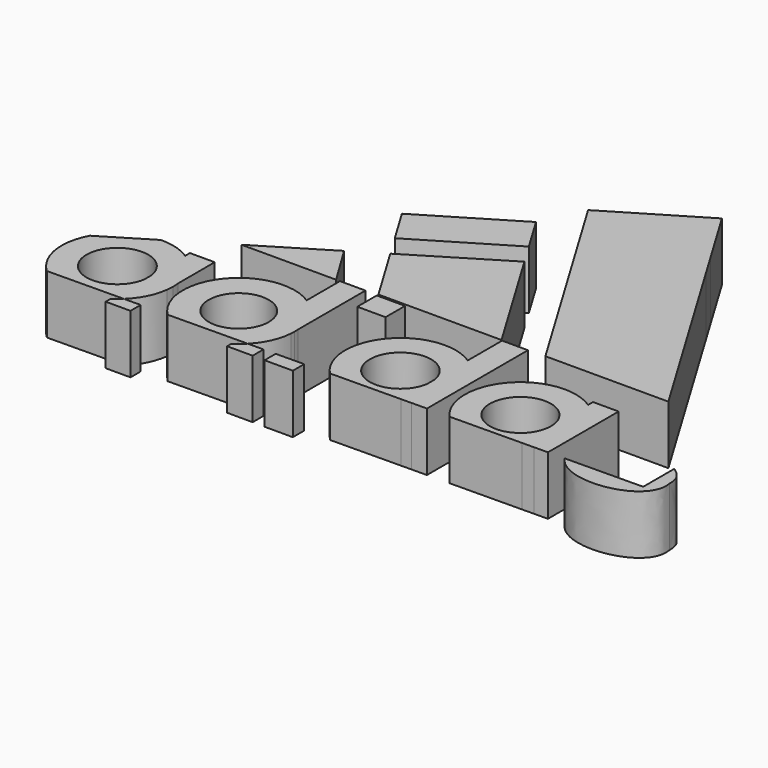
from build123d import *

# Parameters (mm, degrees)
F1_DEPTH = 7.62
F0_R     = 3.9071612502
F0_R_2   = 3.9693222288
F0_W     = 3.6783010967
F0_H     = 3.1684441492


with BuildPart() as f1:
    # F0 (on Top) → F1 (new body)
    with BuildSketch(Plane.XY):
        Polygon((-54.6120963991, 18.8028495759), (-57.9414791113, 24.2596925711), (-66.9205742951, 18.8028495759), align=None)
    extrude(amount=F1_DEPTH)


with BuildPart() as f1b:
    # F0 (on Top) → F1, piece 2 (new body)
    with BuildSketch(Plane.XY):
        Polygon((-58.4635436535, 34.3171171844), (-55.6590456115, 29.6528524318), (-43.8780021033, 36.7234046998), (-46.6844625771, 41.399564594), align=None)
    extrude(amount=F1_DEPTH)


with BuildPart() as f1c:
    # F0 (on Top) → F1, piece 3 (new body)
    with BuildSketch(Plane.XY):
        Polygon((-42.1554631157, 33.8532884785), (-53.8949323829, 26.718890265), (-49.2192299373, 18.9425560391), (-33.2065857947, 18.9425560391), align=None)
    extrude(amount=F1_DEPTH)


with BuildPart() as f1d:
    # F0 (on Top) → F1, piece 4 (new body)
    with BuildSketch(Plane.XY):
        with BuildLine():
            ThreePointArc((-69.8677301407, 13.3297108985), (-71.8363877974, 14.2310348582), (-73.9834488266, 14.5105465515))
            Line((-73.9834488266, 14.5105465515), (-80.197720877, 10.7339625846))
            ThreePointArc((-80.197720877, 10.7339625846), (-80.9859151306, 6.0900592734), (-78.7530233725, 1.9426163816))
            Line((-78.7530233725, 1.9426163816), (-69.8677301407, 2.0325591908))
            Line((-69.8677301407, 2.0325591908), (-69.8677301407, 6.657484785))
            ThreePointArc((-69.8677301407, 6.657484785), (-77.8484436742, 7.2651901282), (-69.8677301407, 7.8728954714))
            Line((-69.8677301407, 7.8728954714), (-69.8677301407, 13.3297108985))
        make_face()
        with BuildLine():
            Line((-69.8677301407, 14.1047984362), (-69.8677301407, 13.3297108985))
            ThreePointArc((-69.8677301407, 13.3297108985), (-67.6845522307, 11.0979247886), (-66.6428804398, 8.1547878725))
            Line((-66.6428804398, 8.1547878725), (-66.6428804398, 14.1047984362))
            Line((-66.6428804398, 14.1047984362), (-69.8677301407, 14.1047984362))
        make_face()
        with BuildLine():
            ThreePointArc((-66.6428804398, 8.1547878725), (-67.6845522307, 11.0979247886), (-69.8677301407, 13.3297108985))
            Line((-69.8677301407, 13.3297108985), (-69.8677301407, 7.8728954714))
            ThreePointArc((-69.8677301407, 7.8728954714), (-69.833040775, 7.5699224451), (-69.821455358, 7.2651901282))
            ThreePointArc((-69.821455358, 7.2651901282), (-69.833040775, 6.9604578114), (-69.8677301407, 6.657484785))
            Line((-69.8677301407, 6.657484785), (-69.8677301407, 2.0325591908))
            Line((-69.8677301407, 2.0325591908), (-68.810137273, 2.0432648447))
            ThreePointArc((-68.810137273, 2.0432648447), (-67.3537989415, 4.0229796207), (-66.6428804398, 6.375592384))
            Line((-66.6428804398, 6.375592384), (-66.6428804398, 8.1547878725))
        make_face()
        with BuildLine():
            ThreePointArc((-66.5880714472, 7.2651901282), (-66.6017866739, 7.7108324097), (-66.6428804398, 8.1547878725))
            Line((-66.6428804398, 8.1547878725), (-66.6428804398, 6.375592384))
            ThreePointArc((-66.6428804398, 6.375592384), (-66.6017866739, 6.8195478467), (-66.5880714472, 7.2651901282))
        make_face()
        with BuildLine():
            ThreePointArc((-69.821455358, 7.2651901282), (-69.833040775, 7.5699224451), (-69.8677301407, 7.8728954714))
            Line((-69.8677301407, 7.8728954714), (-69.8677301407, 6.657484785))
            ThreePointArc((-69.8677301407, 6.657484785), (-69.833040775, 6.9604578114), (-69.821455358, 7.2651901282))
        make_face()
    extrude(amount=F1_DEPTH)


with BuildPart() as f1e:
    # F0 (on Top) → F1, piece 5 (new body)
    with BuildSketch(Plane.XY):
        Polygon((-27.9197386264, 46.3009719113), (-39.6823539035, 39.2414795949), (-37.9737712473, 36.3946175894), (-26.25028293, 43.5193037403), align=None)
        Polygon((-44.1911518574, 46.7540957034), (-39.6823539035, 39.2414795949), (-27.9197386264, 46.3009719113), (-32.4285365804, 53.8135880197), align=None)
        Polygon((-26.25028293, 43.5193037403), (-37.9737712473, 36.3946175894), (-27.4996809606, 18.9425560391), (-11.5002160892, 18.9425560391), align=None)
    extrude(amount=F1_DEPTH)


with BuildPart() as f1f:
    # F0 (on Top) → F1, piece 6 (new body)
    with BuildSketch(Plane.XY):
        with BuildLine():
            ThreePointArc((-54.1104190052, 13.3848092535), (-63.7170999248, 11.8183650375), (-63.1665728512, 2.1003927329))
            Line((-63.1665728512, 2.1003927329), (-54.1104190052, 2.1920651062))
            Line((-54.1104190052, 2.1920651062), (-54.1104190052, 13.3848092535))
        make_face()
        with Locations((-58.0436183297, 7.2651901282)):
            Circle(F0_R, mode=Mode.SUBTRACT)
        with BuildLine():
            Line((-54.1104190052, 18.8028495759), (-54.1104190052, 13.3848092535))
            ThreePointArc((-54.1104190052, 13.3848092535), (-51.7988275156, 10.9964610717), (-50.790913403, 7.8291638969))
            Line((-50.790913403, 7.8291638969), (-50.790913403, 18.8028495759))
            Line((-50.790913403, 18.8028495759), (-54.1104190052, 18.8028495759))
        make_face()
        with BuildLine():
            ThreePointArc((-50.790913403, 7.8291638969), (-51.7988275156, 10.9964610717), (-54.1104190052, 13.3848092535))
            Line((-54.1104190052, 13.3848092535), (-54.1104190052, 2.1920651062))
            Line((-54.1104190052, 2.1920651062), (-52.8171613103, 2.2051563151))
            ThreePointArc((-52.8171613103, 2.2051563151), (-51.4114233914, 4.276246257), (-50.790913403, 6.7012163595))
            Line((-50.790913403, 6.7012163595), (-50.790913403, 7.8291638969))
        make_face()
        with BuildLine():
            ThreePointArc((-50.7690190167, 7.2651901282), (-50.7744946741, 7.5473894266), (-50.790913403, 7.8291638969))
            Line((-50.790913403, 7.8291638969), (-50.790913403, 6.7012163595))
            ThreePointArc((-50.790913403, 6.7012163595), (-50.7744946741, 6.9829908299), (-50.7690190167, 7.2651901282))
        make_face()
    extrude(amount=F1_DEPTH)


with BuildPart() as f1g:
    # F0 (on Top) → F1, piece 7 (new body)
    with BuildSketch(Plane.XY):
        with BuildLine():
            ThreePointArc((-52.8171613103, 2.2051563151), (-53.433248893, 1.6380870705), (-54.1104190052, 1.145571003))
            Line((-54.1104190052, 1.145571003), (-54.1104190052, 0.4571469035))
            Line((-54.1104190052, 0.4571469035), (-50.790913403, 0.4571469035))
            Line((-50.790913403, 0.4571469035), (-50.790913403, 2.2256673353))
            Line((-50.790913403, 2.2256673353), (-52.8171613103, 2.2051563151))
        make_face()
    extrude(amount=F1_DEPTH)


with BuildPart() as f1h:
    # F0 (on Top) → F1, piece 8 (new body)
    with BuildSketch(Plane.XY):
        with BuildLine():
            ThreePointArc((-68.810137273, 2.0432648447), (-69.319238061, 1.5972458978), (-69.8677301407, 1.200669358))
            Line((-69.8677301407, 1.200669358), (-69.8677301407, 0.4053486628))
            Line((-69.8677301407, 0.4053486628), (-66.6428804398, 0.4053486628))
            Line((-66.6428804398, 0.4053486628), (-66.6428804398, 2.0652032504))
            Line((-66.6428804398, 2.0652032504), (-68.810137273, 2.0432648447))
        make_face()
    extrude(amount=F1_DEPTH)


with BuildPart() as f1i:
    # F0 (on Top) → F1, piece 9 (new body)
    with BuildSketch(Plane.XY):
        Polygon((-45.5409288406, 2.2788111481), (-49.2192299373, 2.2415769539), (-49.2192299373, 0.4300079017), (-45.5409288406, 0.4300079017), align=None)
    extrude(amount=F1_DEPTH)


with BuildPart() as f1j:
    # F0 (on Top) → F1, piece 10 (new body)
    with BuildSketch(Plane.XY):
        with BuildLine():
            add(Edge.make_bspline(
                [(-0.1574168564, 4.985621199), (-0.1131827791, 6.2999939449), (-0.7987933683, 7.1600216499), (-1.7971183406, 7.7627462702)],
                knots=[0, 0, 0, 0, 2.8581671617, 2.8581671617, 2.8581671617, 2.8581671617], degree=3))
            Line((-1.7971183406, 7.7627462702), (-1.7971183406, 2.7216149028))
            Line((-1.7971183406, 2.7216149028), (-11.9253362085, 2.6190903891))
            add(Edge.make_bspline(
                [(-11.9253362085, 2.6190903891), (-9.1467564623, -1.6533627287), (0.8026806645, 0.0011403924), (-0.1574168564, 4.985621199)],
                knots=[1.6292148337, 1.6292148337, 1.6292148337, 1.6292148337, 12.4734198375, 12.4734198375, 12.4734198375, 12.4734198375], degree=3))
        make_face()
    extrude(amount=F1_DEPTH)


with BuildPart() as f1k:
    # F0 (on Top) → F1, piece 11 (new body)
    with BuildSketch(Plane.XY):
        with BuildLine():
            ThreePointArc((-33.0688804388, 13.2829963894), (-42.5337962649, 11.8763615852), (-42.229529747, 2.3123313179))
            Line((-42.229529747, 2.3123313179), (-33.0688804388, 2.4050614633))
            Line((-33.0688804388, 2.4050614633), (-33.0688804388, 6.6275104705))
            ThreePointArc((-33.0688804388, 6.6275104705), (-41.0053996041, 7.2651901282), (-33.0688804388, 7.902869786))
            Line((-33.0688804388, 7.902869786), (-33.0688804388, 13.2829963894))
        make_face()
        with BuildLine():
            Line((-33.0688804388, 18.8656765968), (-33.0688804388, 13.2829963894))
            ThreePointArc((-33.0688804388, 13.2829963894), (-30.6821030987, 10.6852589728), (-29.8171898923, 7.2651901282))
            ThreePointArc((-29.8171898923, 7.2651901282), (-30.3028664009, 4.6666608213), (-31.6943216201, 2.4189756559))
            Line((-31.6943216201, 2.4189756559), (-29.7021493316, 2.4391417402))
            Line((-29.7021493316, 2.4391417402), (-29.7021493316, 18.8656765968))
            Line((-29.7021493316, 18.8656765968), (-33.0688804388, 18.8656765968))
        make_face()
        with BuildLine():
            ThreePointArc((-29.8171898923, 7.2651901282), (-30.6821030987, 10.6852589728), (-33.0688804388, 13.2829963894))
            Line((-33.0688804388, 13.2829963894), (-33.0688804388, 7.902869786))
            ThreePointArc((-33.0688804388, 7.902869786), (-33.0304740594, 7.5850574725), (-33.0176444577, 7.2651901282))
            ThreePointArc((-33.0176444577, 7.2651901282), (-33.0304740594, 6.945322784), (-33.0688804388, 6.6275104705))
            Line((-33.0688804388, 6.6275104705), (-33.0688804388, 2.4050614633))
            Line((-33.0688804388, 2.4050614633), (-31.6943216201, 2.4189756559))
            ThreePointArc((-31.6943216201, 2.4189756559), (-30.3028664009, 4.6666608213), (-29.8171898923, 7.2651901282))
        make_face()
        with BuildLine():
            ThreePointArc((-33.0176444577, 7.2651901282), (-33.0304740594, 7.5850574725), (-33.0688804388, 7.902869786))
            Line((-33.0688804388, 7.902869786), (-33.0688804388, 6.6275104705))
            ThreePointArc((-33.0688804388, 6.6275104705), (-33.0304740594, 6.945322784), (-33.0176444577, 7.2651901282))
        make_face()
    extrude(amount=F1_DEPTH)


with BuildPart() as f1l:
    # F0 (on Top) → F1, piece 12 (new body)
    with BuildSketch(Plane.XY):
        with BuildLine():
            Line((-15.9099875813, 2.578755115), (-14.0899363905, 2.5971788758))
            Line((-14.0899363905, 2.5971788758), (-14.0899363905, 14.0935815871))
            Line((-14.0899363905, 14.0935815871), (-17.416972667, 14.0935815871))
            Line((-17.416972667, 14.0935815871), (-17.416972667, 13.2860199104))
            ThreePointArc((-17.416972667, 13.2860199104), (-15.0424605066, 10.6824550648), (-14.182717371, 7.2651901282))
            ThreePointArc((-14.182717371, 7.2651901282), (-14.628280923, 4.7678848048), (-15.9099875813, 2.578755115))
        make_face()
        with BuildLine():
            Line((-17.416972667, 2.5635004161), (-15.9099875813, 2.578755115))
            ThreePointArc((-15.9099875813, 2.578755115), (-14.628280923, 4.7678848048), (-14.182717371, 7.2651901282))
            ThreePointArc((-14.182717371, 7.2651901282), (-15.0424605066, 10.6824550648), (-17.416972667, 13.2860199104))
            Line((-17.416972667, 13.2860199104), (-17.416972667, 2.5635004161))
        make_face()
        with BuildLine():
            ThreePointArc((-17.416972667, 13.2860199104), (-26.8585548081, 11.997439908), (-26.8019732469, 2.4684992389))
            Line((-26.8019732469, 2.4684992389), (-17.416972667, 2.5635004161))
            Line((-17.416972667, 2.5635004161), (-17.416972667, 13.2860199104))
        make_face()
        with Locations((-21.4039776474, 7.2651901282)):
            Circle(F0_R_2, mode=Mode.SUBTRACT)
    extrude(amount=F1_DEPTH)


with BuildPart() as f1m:
    # F0 (on Top) → F1, piece 13 (new body)
    with BuildSketch(Plane.XY):
        with Locations((-47.380079389, 17.0888998546)):
            Rectangle(F0_W, F0_H)
    extrude(amount=F1_DEPTH)


solid = Compound([f1.part, f1b.part, f1c.part, f1d.part, f1e.part, f1f.part, f1g.part, f1h.part, f1i.part, f1j.part, f1k.part, f1l.part, f1m.part])
